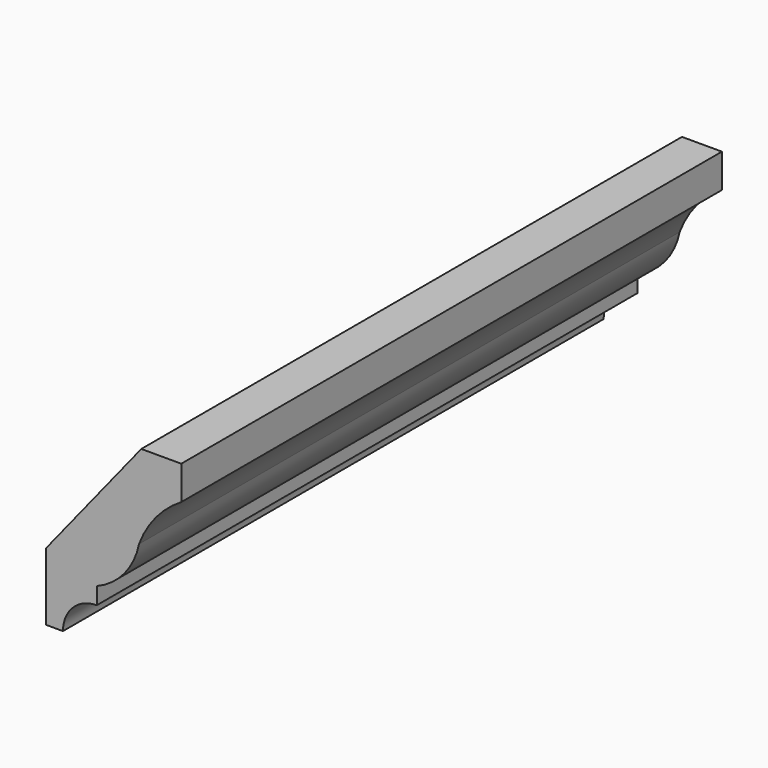
from build123d import *

# Parameters (mm, degrees)
F1_DEPTH = 127


# Not quite as in the source:
# - ends of sketch curves that miss each other by under 0.0002 mm in the source are joined


with BuildPart() as f1:
    # F0 (on Front) → F1 (new body)
    with BuildSketch(Plane.XZ):
        with BuildLine():
            Line((12.7009144, 17.46377), (5.1931316, 17.46377))
            Line((5.1931316, 17.46377), (-12.7009144, -4.7628302))
            Line((-12.7009144, -4.7628302), (-12.7009144, -17.4637446))
            Line((-12.7009144, -17.4637446), (-9.5256858, -17.4637446))
            ThreePointArc((-9.5256858, -17.4637446), (-7.6656799498, -12.9732932502), (-3.1752286, -11.1132874))
            Line((-3.1752286, -11.1132874), (-3.1752286, -7.9380588))
            ThreePointArc((-3.1752286, -7.9380588), (1.9969533726, -4.1778410439), (4.7628402227, 1.5876249697))
            ThreePointArc((4.7628402227, 1.5876249697), (7.9251663957, 7.0227258488), (12.7009100211, 11.1133200969))
            Line((12.7009100211, 11.1133200969), (12.7009144, 17.46377))
        make_face()
    extrude(amount=F1_DEPTH)


solid = f1.part
